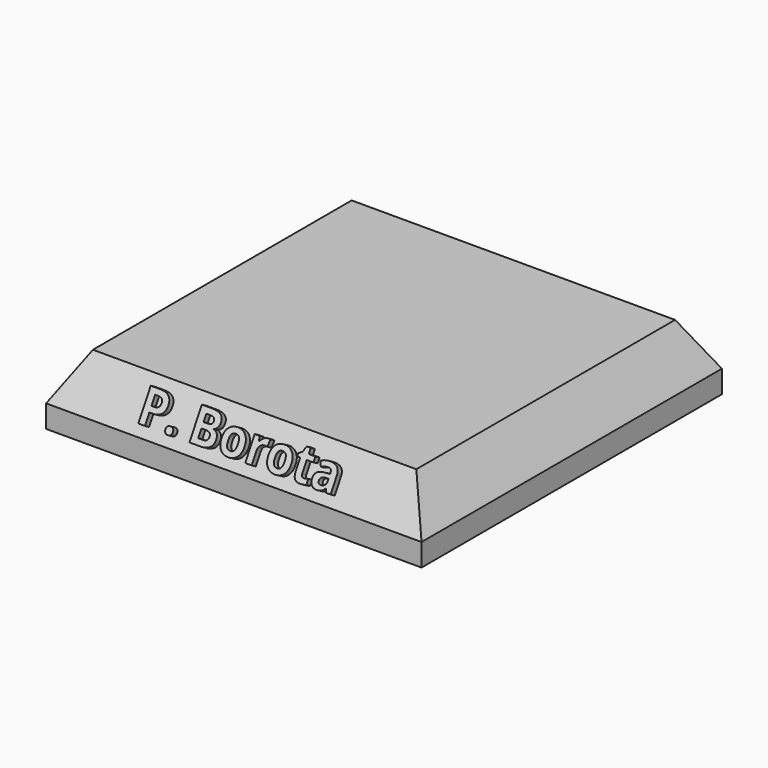
from build123d import *

# Parameters (mm, degrees)
F0_W         = 50
F0_H         = 50
F1_DEPTH     = 9
F2_SIZE2     = 3.4641016151
F2_SIZE      = 6
F3_TEXT_SIZE = 5.8048629074
F4_DEPTH     = 0.8


# Not quite as in the source:
# - Text() gives the source's letters only with a copy of the font that has no kerning and outlines rounded to 1/6400 em; it was checked with that copy


with BuildPart() as f1:
    # F0 (on Top) → F1 (new body)
    with BuildSketch(Plane.XY):
        Rectangle(F0_W, F0_H)
    extrude(amount=F1_DEPTH)

    # F2
    f2_edges = [f1.edges().sort_by_distance(p)[0] for p in [
        (0, 25, 9),
        (-25, 0, 9),
        (0, -25, 9),
        (25, 0, 9),
    ]]
    chamfer(f2_edges, length=F2_SIZE, length2=F2_SIZE2)

    # F3 (on face) → F4 (join)
    with BuildSketch(Plane(origin=(0, -20.0490381057, 11.5753175473), x_dir=(1, 0, 0), z_dir=(0, -0.8660254038, 0.5))):
        with Locations((-13.2495995862, -8.4936656916)):
            Text('P. Borota', F3_TEXT_SIZE, font='Open Sans', font_style=FontStyle.BOLD, text_align=(TextAlign.LEFT, TextAlign.BOTTOM))
    extrude(amount=F4_DEPTH)


solid = f1.part
